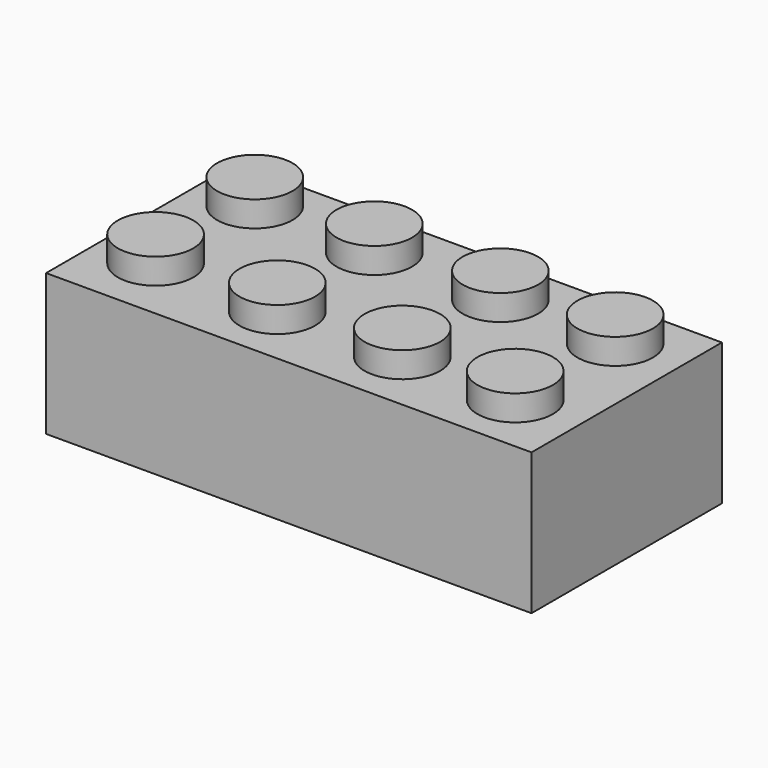
from build123d import *

# Parameters (mm, degrees)
F0_W     = 31.3436
F0_H     = 9.144
F1_DEPTH = 15.367
F2_R     = 2.4384
F3_DEPTH = 1.651
F4_T     = -1.1938
F5_R     = 3.2258
F6_DEPTH = 7.88406
F7_R     = 2.4384
F8_DEPTH = 8.37132


# Not quite as in the source:
# - the program builds the solid bodies; features that only make, move or delete a surface that nothing else refers to are left out


with BuildPart() as f1:
    # F0 (on Front) → F1 (new body)
    with BuildSketch(Plane.XZ):
        Rectangle(F0_W, F0_H)
    extrude(amount=F1_DEPTH)

    # F2 (on face) → F3 (join)
    with BuildSketch(Plane.XY.offset(4.572)):
        with Locations((-12.0193809271, -3.087217221)):
            Circle(F2_R)
        with Locations((-4.1364012286, -3.2935778145)):
            Circle(F2_R)
        with Locations((4.0354835801, -3.33484984)):
            Circle(F2_R)
        with Locations((11.5470141172, -3.4586666152)):
            Circle(F2_R)
        with Locations((11.4644700661, -11.4241903648)):
            Circle(F2_R)
        with Locations((4.0767556056, -11.3003747538)):
            Circle(F2_R)
        with Locations((-3.9300406352, -11.3829188049)):
            Circle(F2_R)
        with Locations((-12.0193809271, -11.094013229)):
            Circle(F2_R)
    extrude(amount=F3_DEPTH)

    # F4
    f4_openings = [f1.faces().sort_by_distance(p)[0] for p in [
        (0, -7.6835, -4.572),
    ]]
    offset(amount=F4_T, openings=f4_openings, kind=Kind.INTERSECTION)

    # F5 (on face) → F6 (join)
    with BuildSketch(Plane(origin=(0, 0, 3.3782), x_dir=(1, 0, 0), z_dir=(0, 0, -1))):
        with Locations((-8.1251291558, 7.3120272718)):
            Circle(F5_R)
        with Locations((0, 7.1467519738)):
            Circle(F5_R)
        with Locations((7.7412822284, 7.3671187274)):
            Circle(F5_R)
    extrude(amount=F6_DEPTH)

    # F7 (on face) → F8 (cut)
    with BuildSketch(Plane(origin=(0, 0, -4.50586), x_dir=(1, 0, 0), z_dir=(0, 0, -1))):
        with Locations((-8.1251291558, 7.3120272718)):
            Circle(F7_R)
        with Locations((-0.012788114, 7.1699875407)):
            Circle(F7_R)
        with Locations((7.7589382418, 7.4168494903)):
            Circle(F7_R)
    extrude(amount=-F8_DEPTH, mode=Mode.SUBTRACT)


solid = f1.part
